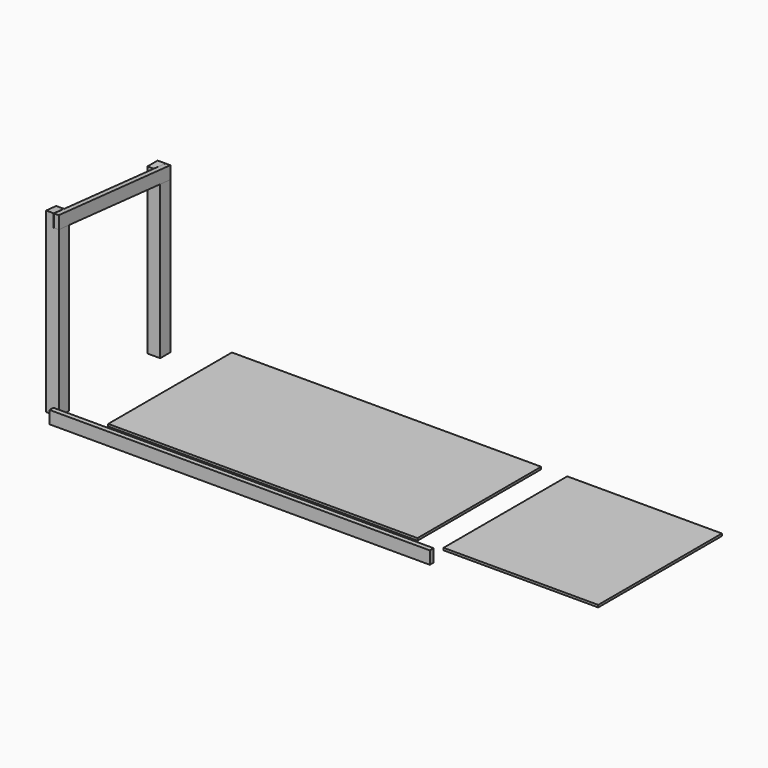
from build123d import *

# Parameters (mm, degrees)
F0_W      = 100
F0_H      = 100
F1_DEPTH  = 1400
F2_DEPTH  = 1300
F3_W      = 38
F3_H      = 100
F4_DEPTH  = 3000
F5_W      = 2440
F5_H      = 1220
F6_DEPTH  = 18
F5_W_2    = 1220
F8_DEPTH  = 100
F9_DEPTH  = 40
F10_DEPTH = 38


# Not quite as in the source:
# - a feature names something its author has since deleted; it is built from what else it names


with BuildPart() as f1:
    # F0 (on Top) → F1 (new body)
    with BuildSketch(Plane.XY):
        with Locations((-68.3726489544, 50)):
            Rectangle(F0_W, F0_H)
    extrude(amount=F1_DEPTH)

    # F7 (on face) → F8 (cut, through all)
    with BuildSketch(Plane.YZ.offset(-18.3726489544)):
        Polygon((0, 1400), (100, 1390.9090909091), (100, 1400), align=None)
    extrude(amount=-F8_DEPTH, mode=Mode.SUBTRACT)


with BuildPart() as f2:
    # F0 (on Top) → F2 (new body)
    with BuildSketch(Plane.XY):
        with Locations((-68.3726489544, 1050)):
            Rectangle(F0_W, F0_H)
    extrude(amount=F2_DEPTH)


with BuildPart() as f4:
    # F3 (on Right) → F4 (new body)
    with BuildSketch(Plane.YZ):
        with Locations((-95.0890891392, 50)):
            Rectangle(F3_W, F3_H)
    extrude(amount=F4_DEPTH)


with BuildPart() as f6:
    # F5 (on Top) → F6 (new body)
    with BuildSketch(Plane.XY):
        with Locations((1520.0716269016, 699.3870592117)):
            Rectangle(F5_W, F5_H)
    extrude(amount=F6_DEPTH)


with BuildPart() as f6b:
    # F5 (on Top) → F6, piece 2 (new body)
    with BuildSketch(Plane.XY):
        with Locations((3555.6486701965, 699.3870592117)):
            Rectangle(F5_W_2, F5_H)
    extrude(amount=F6_DEPTH)


with BuildPart() as f9_tool:
    # F7 (on face) → F9 (new body)
    with BuildSketch(Plane.YZ.offset(-18.3726489544)):
        Polygon((0, 1299.5876271165), (100, 1290.4967180256), (100, 1390.9090909091), (0, 1400), align=None)
        Polygon((1000, 1300), (1000, 1208.6785362074), (1100, 1199.5876271165), (1100, 1300), align=None)
    extrude(amount=-F9_DEPTH)


with BuildPart() as f1_1:
    add(f1.part)

    # F9: cut by f9_tool
    add(f9_tool.part, mode=Mode.SUBTRACT)


with BuildPart() as f2_1:
    add(f2.part)

    # F9: cut by f9_tool
    add(f9_tool.part, mode=Mode.SUBTRACT)


with BuildPart() as f10:
    # F7 (on face) → F10 (new body)
    with BuildSketch(Plane.YZ.offset(-18.3726489544)):
        Polygon((0, 1299.5876271165), (100, 1290.4967180256), (100, 1390.9090909091), (0, 1400), align=None)
        Polygon((1000, 1309.0909090909), (1000, 1300), (1100, 1300), align=None)
        Polygon((1000, 1300), (1000, 1208.6785362074), (1100, 1199.5876271165), (1100, 1300), align=None)
        Polygon((100, 1290.4967180256), (1000, 1208.6785362074), (1000, 1300), (1000, 1309.0909090909), (100, 1390.9090909091), align=None)
    extrude(amount=-F10_DEPTH)


solid = Compound([f4.part, f6.part, f6b.part, f1_1.part, f2_1.part, f10.part])
